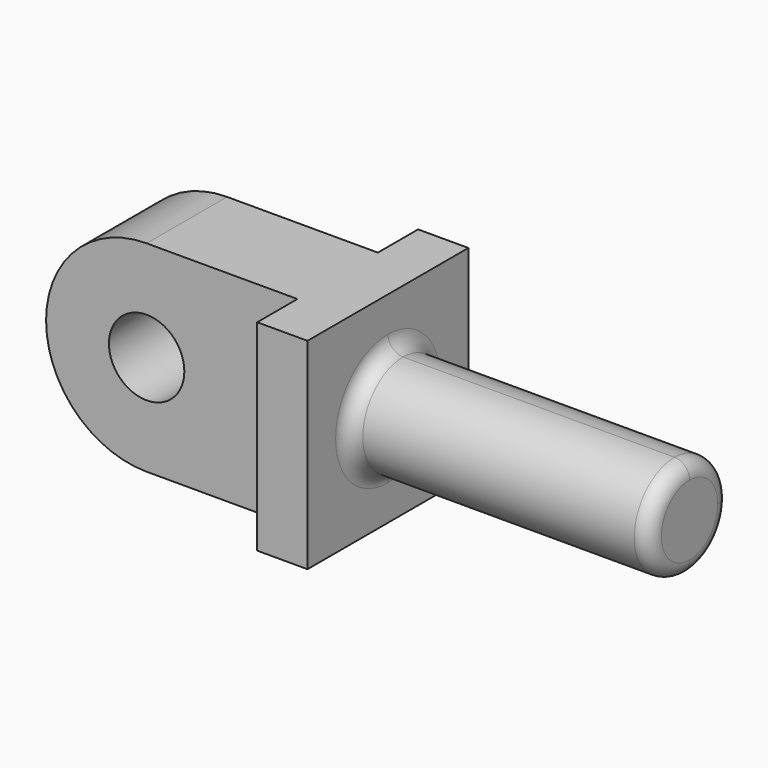
from build123d import *

# Parameters (mm, degrees)
F0_W     = 76.2
F0_H     = 50.8
F1_DEPTH = 50.8
F2_W     = 63.5
F2_H     = 12.7
F3_DEPTH = 177.8
F5_DEPTH = 127
F6_R     = 25.39999
F8_DEPTH = 76.2
F9_R     = 3.81


# Not quite as in the source:
# - a fillet or chamfer is up to 0.001 mm smaller than in the source, because OpenCascade refuses the exact size


with BuildPart() as f1:
    # F0 (on Front) → F1 (new body)
    with BuildSketch(Plane.XZ):
        with Locations((38.1, 25.4)):
            Rectangle(F0_W, F0_H)
    extrude(amount=F1_DEPTH)

    # F2 (on face) → F3 (cut)
    with BuildSketch(Plane.XY.offset(50.8)):
        with Locations((31.75, -6.35)):
            Rectangle(F2_W, F2_H)
        with Locations((31.75, -44.45)):
            Rectangle(F2_W, F2_H)
    extrude(amount=-F3_DEPTH, mode=Mode.SUBTRACT)

    # F4 (on face) → F5 (cut)
    with BuildSketch(Plane.XZ.offset(38.1)):
        with BuildLine():
            ThreePointArc((15.875, 25.4), (25.4, 15.875), (34.925, 25.4))
            ThreePointArc((34.925, 25.4), (25.4, 34.925), (15.875, 25.4))
        make_face()
    extrude(amount=-F5_DEPTH, mode=Mode.SUBTRACT)

    # F6 (radius 25.4 in the source; OpenCascade refuses exactly that, so slightly less here)
    f6_edges = [f1.edges().sort_by_distance(p)[0] for p in [
        (0, -25.4, 0),
        (0, -25.4, 50.8),
    ]]
    fillet(f6_edges, radius=F6_R)

    # F7 (on face) → F8 (join)
    with BuildSketch(Plane.YZ.offset(76.2)):
        with BuildLine():
            ThreePointArc((-12.7, 25.4), (-16.4197438789, 34.3802561211), (-25.4, 38.1))
            Line((-25.4, 38.1), (-25.4, 12.7))
            ThreePointArc((-25.4, 12.7), (-16.4197438789, 16.4197438789), (-12.7, 25.4))
        make_face()
        with BuildLine():
            Line((-25.4, 12.7), (-25.4, 38.1))
            ThreePointArc((-25.4, 38.1), (-38.1, 25.4), (-25.4, 12.7))
        make_face()
    extrude(amount=F8_DEPTH)

    # F9
    f9_edges = [f1.edges().sort_by_distance(p)[0] for p in [
        (152.4, -38.1, 25.4),
        (76.2, -38.1, 25.4),
    ]]
    fillet(f9_edges, radius=F9_R)


solid = f1.part
